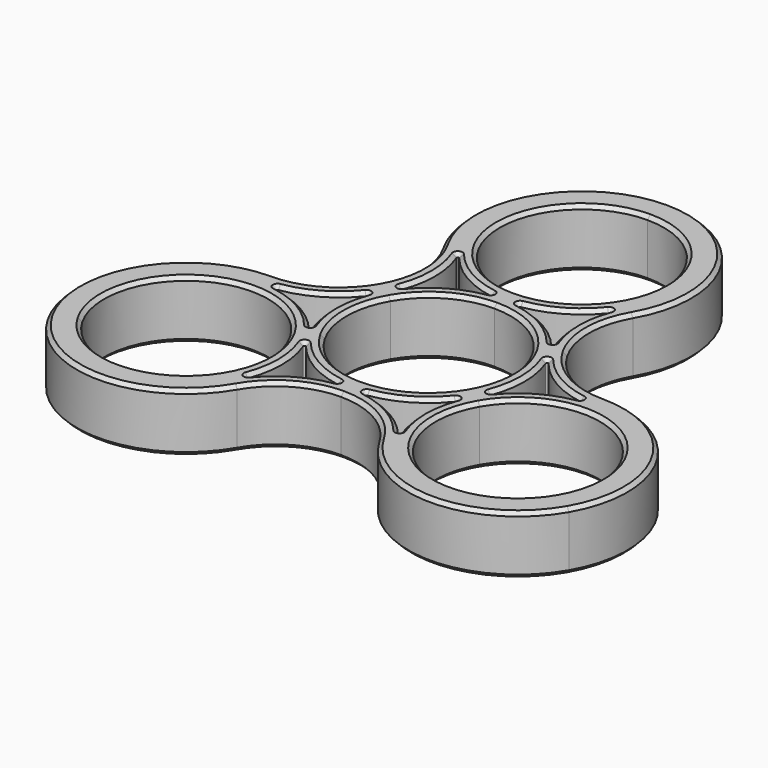
from build123d import *
from build123d import SkipClean  # not in build123d's __all__

# Parameters (mm, degrees)
F1_DEPTH = 8
F3_DEPTH = 8.001
F4_SIZE  = 0.5
F6_COUNT = 3


with BuildPart() as f1:
    # F0 (on Top) → F1 (new body)
    with BuildSketch(Plane.XY):
        with BuildLine():
            ThreePointArc((0, 11.25), (5.625, 9.7427857926), (9.7427857926, 5.625))
            Line((9.7427857926, 5.625), (12.9903810568, 7.5))
            ThreePointArc((12.9903810568, 7.5), (11.4831668493, 13.125), (12.9903810568, 18.75))
            ThreePointArc((12.9903810568, 18.75), (12.9903810568, 33.75), (0, 41.25))
            Line((0, 41.25), (0, 37.5))
            ThreePointArc((0, 37.5), (11.25, 26.25), (0, 15))
            Line((0, 15), (0, 11.25))
        make_face()
    extrude(amount=F1_DEPTH)

    # F2 (on Top) → F3 (cut, through all)
    with BuildSketch(Plane.XY):
        with BuildLine():
            ThreePointArc((10.2291824432, 18.0262872409), (6.5625, 14.8834165753), (2.0073529412, 13.2794117647))
            ThreePointArc((2.0073529412, 13.2794117647), (1.875, 13.125), (2.0073529412, 12.9705882353))
            ThreePointArc((2.0073529412, 12.9705882353), (6.5625, 11.3665834247), (10.2291824432, 8.2237127591))
            ThreePointArc((10.2291824432, 8.2237127591), (10.4290834247, 8.1862976321), (10.496631465, 8.3781245238))
            ThreePointArc((10.496631465, 8.3781245238), (9.6081668493, 13.125), (10.496631465, 17.8718754762))
            ThreePointArc((10.496631465, 17.8718754762), (10.4290834247, 18.0637023679), (10.2291824432, 18.0262872409))
        make_face()
    extrude(amount=F3_DEPTH, mode=Mode.SUBTRACT)

    # F4
    f4_edges = [f1.edges().sort_by_distance(p)[0] for p in [
        (11.483167, 13.125, 8),
        (5.625, 9.742786, 8),
        (5.625, 9.742786, 0),
        (12.990381, 33.75, 0),
        (11.25, 26.25, 8),
        (11.25, 26.25, 0),
        (12.990381, 33.75, 8),
        (11.483167, 13.125, 0),
        (9.608167, 13.125, 8),
        (6.5625, 11.366583, 0),
    ]]
    chamfer(f4_edges, length=F4_SIZE)

    # F5: F1 across plane


with BuildPart() as f1_1:
    add(f1.part, clean=False)
    with SkipClean():  # cleaning this boolean's faces spoils the solid; the shape is the same uncleaned
        add(f1.part.mirror(Plane.YZ), clean=False)

    # F6: F1 ×3 about axis
    f6_axis = Axis((0, 0, 0), (0, 0, -1))


with BuildPart() as f1_2:
    add(f1_1.part, clean=False)
    for i in range(1, F6_COUNT):
        add(f1_1.part.rotate(f6_axis, i * 360 / F6_COUNT), clean=False)


solid = f1_2.part
